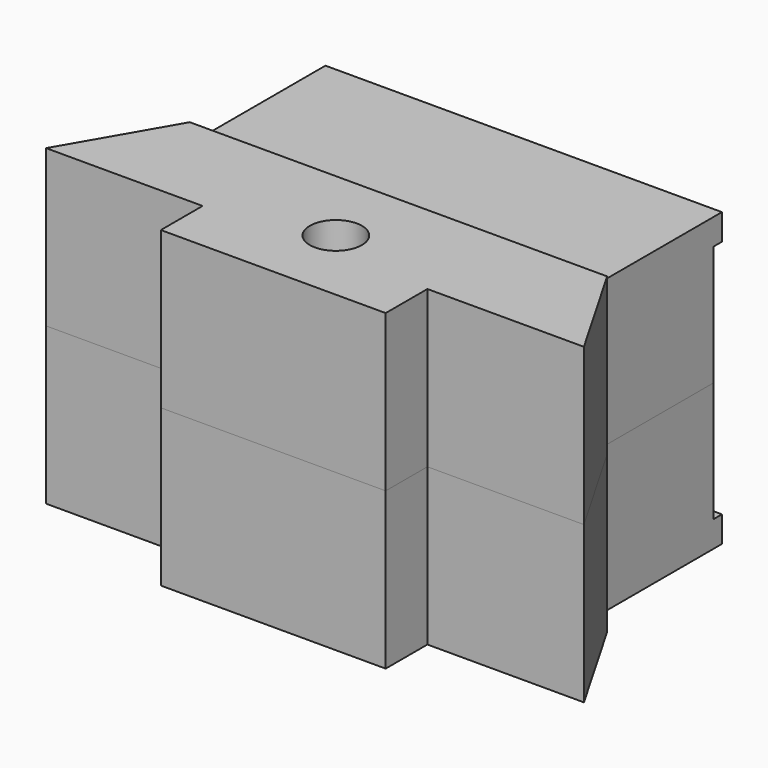
from build123d import *

# Parameters (mm, degrees)
F1_DEPTH = 30
F2_W     = 76
F2_H     = 28
F3_DEPTH = 30
F4_W     = 76
F4_H     = 23
F5_DEPTH = 2
F7_R     = 5
F8_DEPTH = 60
F9_R     = 0.75


# Not quite as in the source:
# - a feature names something its author has since deleted; it is built from what else it names


with BuildPart() as f1:
    # F0 (on Top) → F1 (new body)
    with BuildSketch(Plane.XY):
        Polygon((40, 0), (-40, 0), (-51.5470053838, -20), (-21.5470053838, -20), (-21.5470053838, -30), (21.5470053838, -30), (21.5470053838, -20), (51.5470053838, -20), align=None)
    extrude(amount=F1_DEPTH)

    # F2 (on face) → F3 (join)
    with BuildSketch(Plane(origin=(0, 0, 0), x_dir=(-1, 0, 0), z_dir=(0, 1, 0))):
        with Locations((0, 14)):
            Rectangle(F2_W, F2_H)
    extrude(amount=F3_DEPTH)

    # F4 (on face) → F5 (cut)
    with BuildSketch(Plane(origin=(0, 30, 0), x_dir=(-1, 0, 0), z_dir=(0, 1, 0))):
        with Locations((0, 11.5)):
            Rectangle(F4_W, F4_H)
    extrude(amount=-F5_DEPTH, mode=Mode.SUBTRACT)


with BuildPart() as f6_1:
    # F6: instance of F1
    add(f1.part.mirror(Plane.XY))


with BuildPart() as f8_tool:
    # F7 (on face) → F8 (new body, through all)
    with BuildSketch(Plane.XY.offset(30)):
        with Locations((0, -15)):
            Circle(F7_R)
    extrude(amount=-F8_DEPTH)


with BuildPart() as f1_1:
    add(f1.part)

    # F8: cut by f8_tool
    add(f8_tool.part, mode=Mode.SUBTRACT)


with BuildPart() as f6_1_1:
    add(f6_1.part)

    # F8: cut by f8_tool
    add(f8_tool.part, mode=Mode.SUBTRACT)

    # F9 (on Right) → F10 (revolve, cut)
    with BuildSketch(Plane.YZ):
        with Locations((-10, -30)):
            Circle(F9_R)
    revolve(axis=Axis((0, -15, -32.4979101866), (0, 0, -1)), mode=Mode.SUBTRACT)


solid = Compound([f1_1.part, f6_1_1.part])
